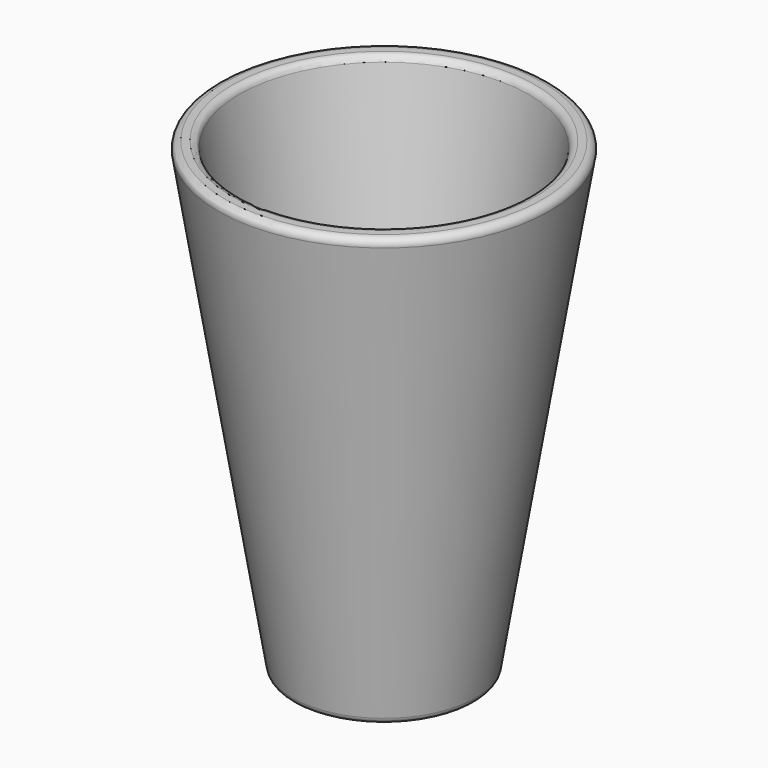
from build123d import *

# Parameters (mm, degrees)
F2_T = -3
F3_R = 1


with BuildPart() as f1:
    # F0 (on Front) → F1 (revolve)
    with BuildSketch(Plane.XZ):
        Polygon((-12.8197669983, 0), (0, 0), (0, 65.9302324057), (-23.5926825553, 65.9302324057), align=None)
    revolve(axis=Axis((0, 0, 32.9651162028), (0, 0, 1)))

    # F2
    f2_openings = [f1.faces().sort_by_distance(p)[0] for p in [
        (0, 0, 65.930232),
    ]]
    offset(amount=F2_T, openings=f2_openings)

    # F3
    f3_edges = [f1.edges().sort_by_distance(p)[0] for p in [
        (23.592683, 0, 65.930232),
        (20.552898, 0, 65.930232),
        (12.819767, 0, 0),
    ]]
    fillet(f3_edges, radius=F3_R)


solid = f1.part
